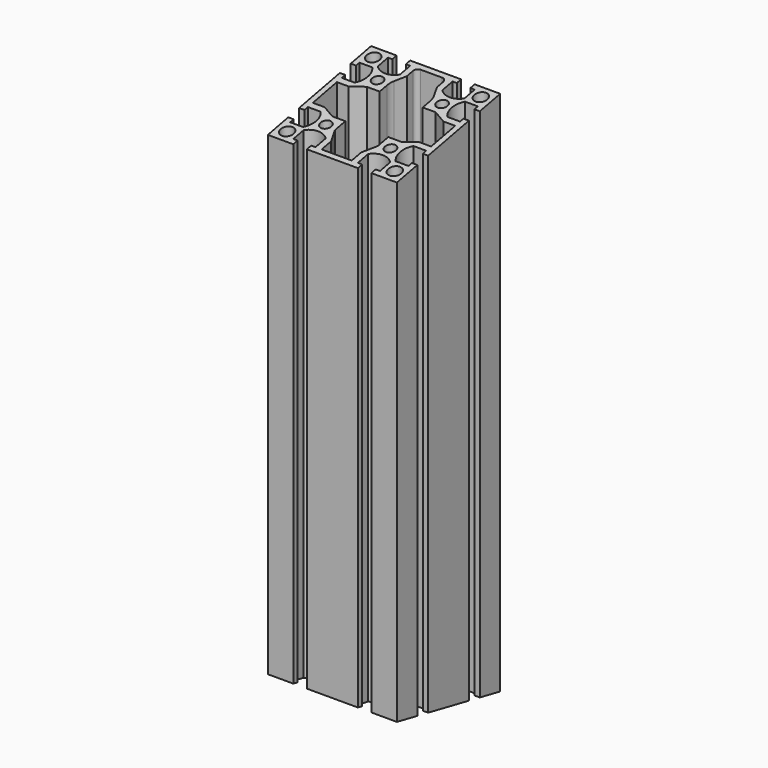
from build123d import *

# Parameters (mm, degrees)
F0_R          = 3
F0_R_2        = 2.5
F1_DEPTH      = 244.595
F2_R          = 2
F3_R          = 7
F5_DEPTH      = 30
F5_DEPTH_BACK = 30


# Not quite as in the source:
# - a feature names something its author has since deleted; it is built from what else it names


with BuildPart() as f1:
    # F0 (on Top) → F1 (new body)
    with BuildSketch(Plane.XY):
        with BuildLine():
            Line((18.15, -30), (30, -30))
            Line((30, -30), (30, -18.15))
            Line((30, -18.15), (27.5, -18.15))
            Line((27.5, -18.15), (27.5, -20.15))
            Line((27.5, -20.15), (21.5477069044, -20.15))
            ThreePointArc((21.5477069044, -20.15), (19.5, -15), (21.5477069044, -9.85))
            Line((21.5477069044, -9.85), (27.5, -9.85))
            Line((27.5, -9.85), (27.5, -11.85))
            Line((27.5, -11.85), (30, -11.85))
            Line((30, -11.85), (30, 11.85))
            Line((30, 11.85), (27.5, 11.85))
            Line((27.5, 11.85), (27.5, 9.85))
            Line((27.5, 9.85), (21.5477069044, 9.85))
            ThreePointArc((21.5477069044, 9.85), (19.5, 15), (21.5477069044, 20.15))
            Line((21.5477069044, 20.15), (27.5, 20.15))
            Line((27.5, 20.15), (27.5, 18.15))
            Line((27.5, 18.15), (30, 18.15))
            Line((30, 18.15), (30, 30))
            Line((30, 30), (18.15, 30))
            Line((18.15, 30), (18.15, 27.5))
            Line((18.15, 27.5), (20.15, 27.5))
            Line((20.15, 27.5), (20.15, 21.5477069044))
            ThreePointArc((20.15, 21.5477069044), (15, 19.5), (9.85, 21.5477069044))
            Line((9.85, 21.5477069044), (9.85, 27.5))
            Line((9.85, 27.5), (11.85, 27.5))
            Line((11.85, 27.5), (11.85, 30))
            Line((11.85, 30), (-11.85, 30))
            Line((-11.85, 30), (-11.85, 27.5))
            Line((-11.85, 27.5), (-9.85, 27.5))
            Line((-9.85, 27.5), (-9.85, 21.5477069044))
            ThreePointArc((-9.85, 21.5477069044), (-15, 19.5), (-20.15, 21.5477069044))
            Line((-20.15, 21.5477069044), (-20.15, 27.5))
            Line((-20.15, 27.5), (-18.15, 27.5))
            Line((-18.15, 27.5), (-18.15, 30))
            Line((-18.15, 30), (-30, 30))
            Line((-30, 30), (-30, 18.15))
            Line((-30, 18.15), (-27.5, 18.15))
            Line((-27.5, 18.15), (-27.5, 20.15))
            Line((-27.5, 20.15), (-21.5477069044, 20.15))
            ThreePointArc((-21.5477069044, 20.15), (-19.5, 15), (-21.5477069044, 9.85))
            Line((-21.5477069044, 9.85), (-27.5, 9.85))
            Line((-27.5, 9.85), (-27.5, 11.85))
            Line((-27.5, 11.85), (-30, 11.85))
            Line((-30, 11.85), (-30, -11.85))
            Line((-30, -11.85), (-27.5, -11.85))
            Line((-27.5, -11.85), (-27.5, -9.85))
            Line((-27.5, -9.85), (-21.5477069044, -9.85))
            ThreePointArc((-21.5477069044, -9.85), (-19.5, -15), (-21.5477069044, -20.15))
            Line((-21.5477069044, -20.15), (-27.5, -20.15))
            Line((-27.5, -20.15), (-27.5, -18.15))
            Line((-27.5, -18.15), (-30, -18.15))
            Line((-30, -18.15), (-30, -30))
            Line((-30, -30), (-18.15, -30))
            Line((-18.15, -30), (-18.15, -27.5))
            Line((-18.15, -27.5), (-20.15, -27.5))
            Line((-20.15, -27.5), (-20.15, -21.5477069044))
            ThreePointArc((-20.15, -21.5477069044), (-15, -19.5), (-9.85, -21.5477069044))
            Line((-9.85, -21.5477069044), (-9.85, -27.5))
            Line((-9.85, -27.5), (-11.85, -27.5))
            Line((-11.85, -27.5), (-11.85, -30))
            Line((-11.85, -30), (11.85, -30))
            Line((11.85, -30), (11.85, -27.5))
            Line((11.85, -27.5), (9.85, -27.5))
            Line((9.85, -27.5), (9.85, -21.5477069044))
            ThreePointArc((9.85, -21.5477069044), (15, -19.5), (20.15, -21.5477069044))
            Line((20.15, -21.5477069044), (20.15, -27.5))
            Line((20.15, -27.5), (18.15, -27.5))
            Line((18.15, -27.5), (18.15, -30))
        make_face()
        with Locations((-25, -25)):
            Circle(F0_R, mode=Mode.SUBTRACT)
        with Locations((-15, -15)):
            Circle(F0_R_2, mode=Mode.SUBTRACT)
        with Locations((25, -25)):
            Circle(F0_R, mode=Mode.SUBTRACT)
        with Locations((15, -15)):
            Circle(F0_R_2, mode=Mode.SUBTRACT)
        with Locations((-25, 25)):
            Circle(F0_R, mode=Mode.SUBTRACT)
        with Locations((-15, 15)):
            Circle(F0_R_2, mode=Mode.SUBTRACT)
        Polygon((-7, 22), (-7, 27.5), (0, 27.5), (7, 27.5), (7, 22), (10, 16), (10, 10), (16, 10), (22, 7), (27.5, 7), (27.5, 0), (27.5, -7), (22, -7), (16, -10), (10, -10), (10, -16), (7, -22), (7, -27.5), (0, -27.5), (-7, -27.5), (-7, -22), (-10, -16), (-10, -10), (-16, -10), (-22, -7), (-27.5, -7), (-27.5, 0), (-27.5, 7), (-22, 7), (-16, 10), (-10, 10), (-10, 16), align=None, mode=Mode.SUBTRACT)
        with Locations((15, 15)):
            Circle(F0_R_2, mode=Mode.SUBTRACT)
        with Locations((25, 25)):
            Circle(F0_R, mode=Mode.SUBTRACT)
    extrude(amount=F1_DEPTH)

    # F2
    f2_edges = [f1.edges().sort_by_distance(p)[0] for p in [
        (-7, 27.5, 122.2975),
        (7, 27.5, 122.2975),
    ]]
    fillet(f2_edges, radius=F2_R)

    # F3
    f3_edges = [f1.edges().sort_by_distance(p)[0] for p in [
        (-10, 16, 122.2975),
        (10, 16, 122.2975),
    ]]
    fillet(f3_edges, radius=F3_R)

    # F4 (on Right) → F5 (cut, two sides)
    with BuildSketch(Plane.YZ) as f5_sk:
        Polygon((6.0593712047, -120.3576686088), (30, 0), (-94.0233882431, 24.6697857659), (-117.9640170384, -95.6878828429), align=None)
        Polygon((30, 244.595), (11.5280437604, 337.4597951001), (-122.8815300181, 310.7240685814), (-104.4095737785, 217.8592734812), align=None)
    extrude(amount=-F5_DEPTH, mode=Mode.SUBTRACT)
    extrude(f5_sk.sketch, amount=F5_DEPTH_BACK, mode=Mode.SUBTRACT)


solid = f1.part
